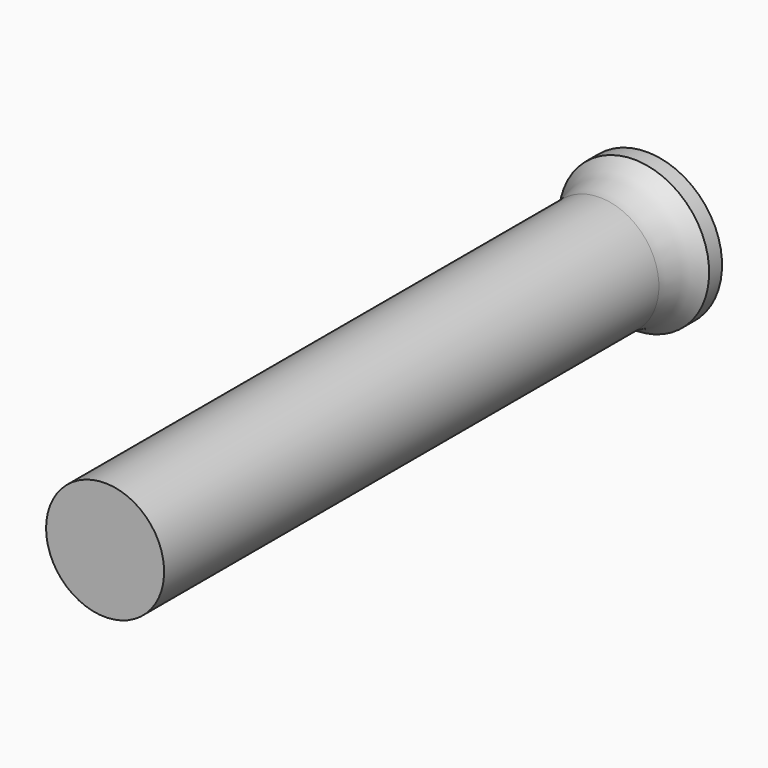
from build123d import *


# Not quite as in the source:
# - a fillet or chamfer that OpenCascade refuses, or shapes differently, is made with other operations: its cross-section is extruded or revolved along the edge and cut away or added


with BuildPart() as f1:
    # F0 (on Top) → F1 (revolve)
    with BuildSketch(Plane.XY):
        Polygon((-4.6482, 0), (0, 0), (0, 6.8579994701), (-3.175, 6.8579994701), (-3.175, 53.34), (-4.6482, 53.34), (-5.9182, 53.34), (-5.9182, 52.07), (-4.6482, 52.07), align=None)
    revolve(axis=Axis((0, 3.4289997351, 0), (0, -1, 0)))

    # F2: fillet of radius 5.08 on 1 edges, made by hand

    # F2_s1 → F2_t2 (revolve)
    with BuildSketch(Plane.XY):
        with BuildLine():
            ThreePointArc((-5.9182, 52.07), (-4.9762951188, 50.5059470592), (-4.6482, 48.7098958349))
            Line((-4.6482, 48.7098958349), (-4.6482, 52.07))
            Line((-4.6482, 52.07), (-5.9182, 52.07))
        make_face()
    revolve(axis=Axis((0, 52.07, 0), (0, -1, 0)))


solid = f1.part
